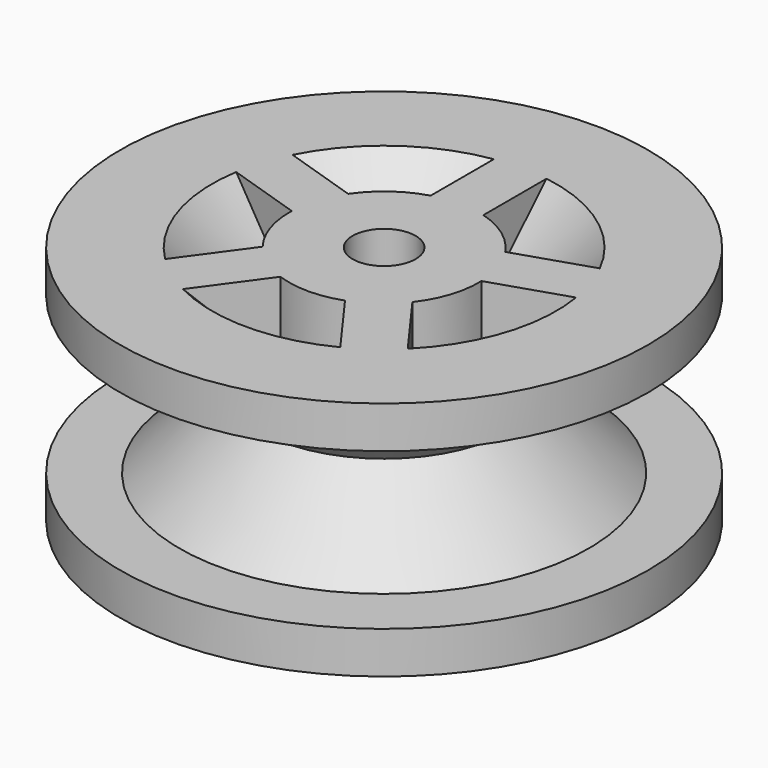
from build123d import *

# Parameters (mm, degrees)
F0_R     = 15.9004
F1_DEPTH = 7.239
F2_R     = 1.89865
F3_DEPTH = 14.479
F6_W     = 3.175
F6_H     = 7.507812879


# Not quite as in the source:
# - a feature names something its author has since deleted; it is built from what else it names


with BuildPart() as f1:
    # F0 (on Top) → F1 (new body, symmetric)
    with BuildSketch(Plane.XY):
        Circle(F0_R)
    extrude(amount=F1_DEPTH, both=True)

    # F2 (on face) → F3 (cut, through all)
    with BuildSketch(Plane.XY.offset(7.239)):
        Circle(F2_R)
    extrude(amount=-F3_DEPTH, mode=Mode.SUBTRACT)

    # F4 (on Right) → F5 (revolve, cut)
    with BuildSketch(Plane.YZ):
        Polygon((18.6176884613, -4.7117), (18.6176884613, 4.7117), (12.3317, 4.7117), (7.62, 0), (12.3317, -4.7117), align=None)
        Polygon((5.715, 2.5851280605), (12.0073856063, 8.8775136668), (5.715, 8.8775136668), align=None)
    revolve(axis=Axis((0, 0, 8.1515284255), (0, 0, 1)), mode=Mode.SUBTRACT)

    # F6 (on face) → F7 (join, up to the next surface of F1)
    with BuildSketch(Plane.XY.offset(7.239)):
        with Locations((0, 7.7054322143)):
            Rectangle(F6_W, F6_H)
        Polygon((-10.4079142205, 5.0509326079), (-11.3890431777, 2.0313281687), (-4.248688816, -0.2887136015), (-3.2675598588, 2.7308908377), align=None)
        Polygon((-8.0199447403, -8.3376906272), (-5.4513157831, -10.2039088032), (-1.0383340959, -4.1299605935), (-3.606963053, -2.2637424175), align=None)
        Polygon((5.4513157831, -10.2039088032), (8.0199447403, -8.3376906272), (3.606963053, -2.2637424175), (1.0383340959, -4.1299605935), align=None)
        Polygon((11.3890431777, 2.0313281687), (10.4079142205, 5.0509326079), (3.2675598588, 2.7308908377), (4.248688816, -0.2887136015), align=None)
    extrude(until=Until.NEXT, dir=(0, 0, -1))


solid = f1.part
